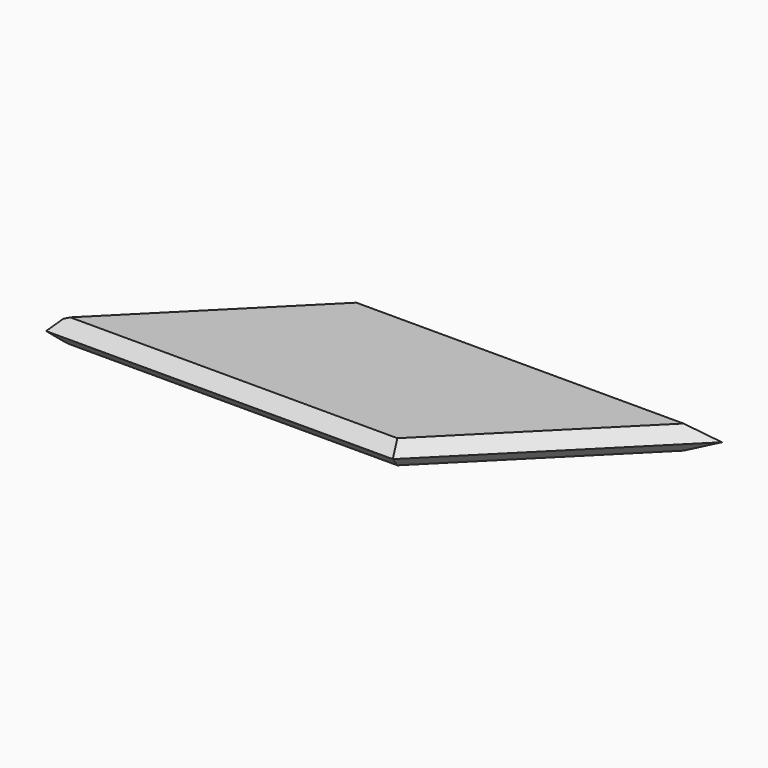
from build123d import *

# Parameters (mm, degrees)
F2_DEPTH    = 3.5
F3_T1_DEPTH = 105.7168298797
F3_T3_DEPTH = 135.7168298797
F3_T5_DEPTH = 105.7168298797
F3_T7_DEPTH = 135.7168298797
F5_W        = 95.1956471843
F5_H        = 46.5
F6_DEPTH    = 2.75
F7_DEPTH    = 25
F9_DEPTH    = 38.4
F10_DEPTH   = 38.4


# Not quite as in the source:
# - a fillet or chamfer that OpenCascade refuses, or shapes differently, is made with other operations: its cross-section is extruded or revolved along the edge and cut away or added


with BuildPart() as f2:
    # F1 (on offset) → F2 (new body)
    with BuildSketch(Plane.XY.offset(3.5)):
        Polygon((11.806184426, -28.2842712475), (32.3819887268, -28.2842712475), (60.6662599742, 0), (88.9505312217, 28.2842712475), (-21.0494687783, 28.2842712475), (-77.6180112732, -28.2842712475), align=None)
    extrude(amount=F2_DEPTH)

    # F3: chamfer of 5 on 4 edges, made by hand

    # F3_s2 → F3_t1 (cut)
    with BuildSketch(Plane(origin=(12.7096736338, 12.7096736338, 0), x_dir=(0, 0, 1), z_dir=(-0.7071067812, -0.7071067812, 0))):
        Polygon((8.5, 34.8842221135), (3.5, 29.8842221135), (3.5, 34.8842221135), align=None)
    extrude(amount=F3_T1_DEPTH, mode=Mode.SUBTRACT)

    # F3_s4 → F3_t3 (cut)
    with BuildSketch(Plane.YZ.offset(-90.476426213)):
        Polygon((-23.2842712475, 3.5), (-28.2842712475, 8.5), (-28.2842712475, 3.5), align=None)
    extrude(amount=F3_T3_DEPTH, mode=Mode.SUBTRACT)

    # F3_s6 → F3_t5 (cut)
    with BuildSketch(Plane(origin=(-7.0434136596, -7.0434136596, 0), x_dir=(0, 0, 1), z_dir=(0.7071067812, 0.7071067812, 0))):
        Polygon((8.5, 42.897523817), (3.5, 37.897523817), (3.5, 42.897523817), align=None)
    extrude(amount=F3_T5_DEPTH, mode=Mode.SUBTRACT)

    # F3_s8 → F3_t7 (cut)
    with BuildSketch(Plane.YZ.offset(-33.9078837181)):
        Polygon((23.2842712475, 3.5), (28.2842712475, 8.5), (28.2842712475, 3.5), align=None)
    extrude(amount=F3_T7_DEPTH, mode=Mode.SUBTRACT)

    # F5 (on face) → F6 (cut)
    with BuildSketch(Plane.XY.offset(7)):
        with Locations((-19.7168718299, -0.4228247255)):
            Rectangle(F5_W, F5_H)
    extrude(amount=-F6_DEPTH, mode=Mode.SUBTRACT)

    # F4 (on face) → F7 (cut)
    with BuildSketch(Plane(origin=(0, 0, 3.5), x_dir=(1, 0, 0), z_dir=(0, 0, -1))):
        Polygon((-24.8950392013, -18.653216398), (-27.3769648583, -30.3716328172), (-13.6225454044, -33.1324383258), (-13.6225454044, -29.2945806164), align=None)
        Polygon((-72.634305031, 14.8857073556), (-60.9158886119, 17.3676330126), (-71.5572528303, 28.6401268095), (-75.3951105397, 28.6401268095), align=None)
    extrude(amount=-F7_DEPTH, mode=Mode.SUBTRACT)


with BuildPart() as f8_1:
    # F8: instance of F2
    add(f2.part.mirror(Plane.XY.offset(7)))

    # F10 (add): a face of the model
    f10_faces = [f8_1.faces().sort_by_distance(p)[0] for p in [
        (27.8809517622, -0.4228247255, 8.375),
    ]]
    extrude(f10_faces, amount=F10_DEPTH)


with BuildPart() as f2_1:
    add(f2.part)

    # F9 (add): a face of the model
    f9_faces = [f2_1.faces().sort_by_distance(p)[0] for p in [
        (27.8809517622, -0.4228247255, 5.625),
    ]]
    extrude(f9_faces, amount=F9_DEPTH)


solid = Compound([f8_1.part, f2_1.part])
